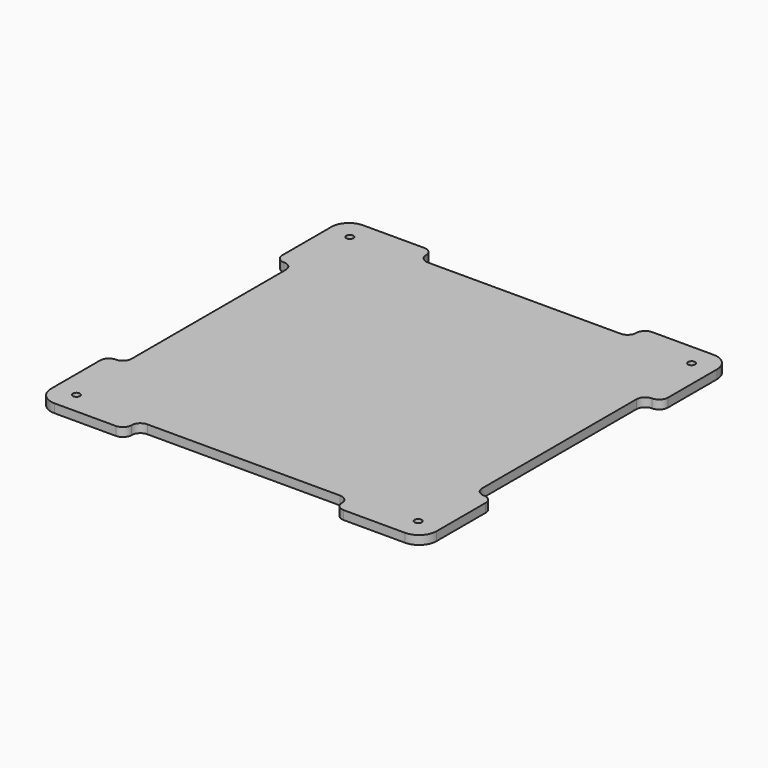
from build123d import *

# Parameters (mm, degrees)
F0_W     = 220
F0_H     = 220
F1_DEPTH = 5
F2_R     = 2
F3_DEPTH = 5.001
F4_W     = 20
F4_H     = 120
F4_W_2   = 120
F4_H_2   = 20
F5_DEPTH = 5.001
F6_R     = 10
F7_R     = 4.99999


# Not quite as in the source:
# - a fillet or chamfer is up to 0.001 mm smaller than in the source, because OpenCascade refuses the exact size


with BuildPart() as f1:
    # F0 (on Top) → F1 (new body)
    with BuildSketch(Plane.XY):
        Rectangle(F0_W, F0_H)
    extrude(amount=F1_DEPTH)

    # F2 (on face) → F3 (cut, through all)
    with BuildSketch(Plane.XY.offset(5)):
        with Locations((-97.5, 97.5)):
            Circle(F2_R)
        with Locations((-97.5, -97.5)):
            Circle(F2_R)
        with Locations((97.5, -97.5)):
            Circle(F2_R)
        with Locations((97.5, 97.5)):
            Circle(F2_R)
    extrude(amount=-F3_DEPTH, mode=Mode.SUBTRACT)

    # F4 (on face) → F5 (cut, through all)
    with BuildSketch(Plane(origin=(0, 0, 0), x_dir=(1, 0, 0), z_dir=(0, 0, -1))):
        with Locations((110, 0)):
            Rectangle(F4_W, F4_H)
        with Locations((0, 110)):
            Rectangle(F4_W_2, F4_H_2)
        with Locations((-110, 0)):
            Rectangle(F4_W, F4_H)
        with Locations((0, -110)):
            Rectangle(F4_W_2, F4_H_2)
    extrude(amount=-F5_DEPTH, mode=Mode.SUBTRACT)

    # F6
    f6_edges = [f1.edges().sort_by_distance(p)[0] for p in [
        (110, -110, 2.5),
        (-110, -110, 2.5),
        (110, 110, 2.5),
        (-110, 110, 2.5),
    ]]
    fillet(f6_edges, radius=F6_R)

    # F7 (radius 5 in the source; OpenCascade refuses exactly that, so slightly less here)
    f7_edges = [f1.edges().sort_by_distance(p)[0] for p in [
        (110, 60, 2.5),
        (100, 60, 2.5),
        (100, -60, 2.5),
        (110, -60, 2.5),
        (60, -100, 2.5),
        (60, -110, 2.5),
        (-60, -100, 2.5),
        (-60, -110, 2.5),
        (-100, -60, 2.5),
        (-110, -60, 2.5),
        (-100, 60, 2.5),
        (-110, 60, 2.5),
        (-60, 100, 2.5),
        (-60, 110, 2.5),
        (60, 100, 2.5),
        (60, 110, 2.5),
    ]]
    fillet(f7_edges, radius=F7_R)


solid = f1.part
